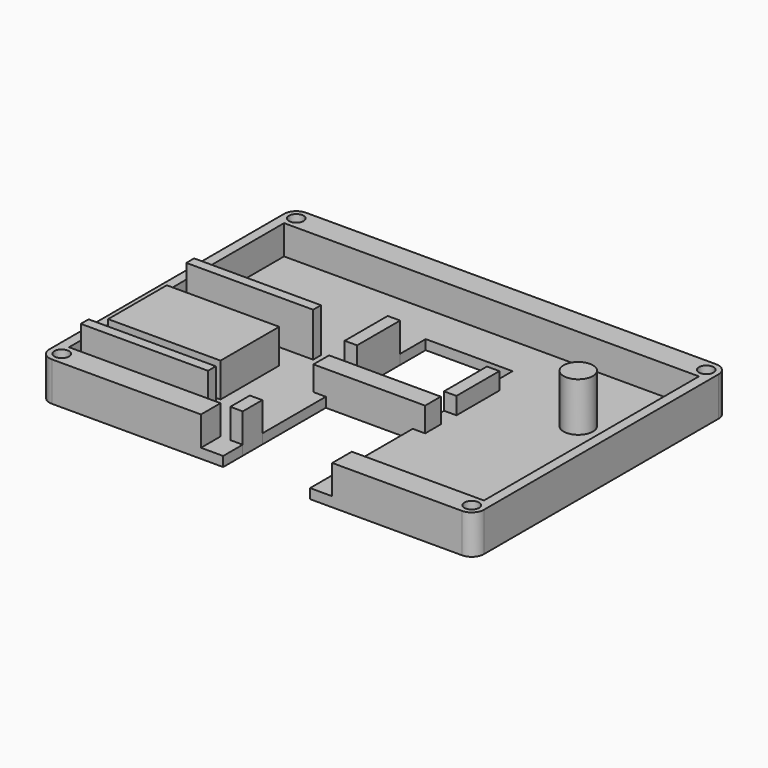
from build123d import *

# Parameters (mm, degrees)
F0_R     = 1.5
F1_DEPTH = 8
F0_W     = 2.54
F0_H     = 11
F0_H_2   = 5
F0_R_2   = 3
F0_H_3   = 16.26
F0_H_4   = 4
F2_DEPTH = 2
F0_W_2   = 23
F0_H_5   = 15
F3_DEPTH = 9
F0_W_3   = 25.9549565881
F0_H_6   = 2
F4_DEPTH = 11
F0_W_4   = 17.78
F5_DEPTH = 7
F6_DEPTH = 5.5
F7_DEPTH = 12


# Not quite as in the source:
# - a feature names something its author has since deleted; it is built from what else it names


with BuildPart() as f1:
    # F0 (on Top) → F1 (new body)
    with BuildSketch(Plane.XY):
        with BuildLine():
            Line((-42.45, 27.5), (42.45, 27.5))
            Line((42.45, 27.5), (42.45, 0.5))
            Line((42.45, 0.5), (42.45, -20.5))
            Line((42.45, -20.5), (42.45, -27.5))
            Line((42.45, -27.5), (15.41, -27.5))
            Line((15.41, -27.5), (15.41, -32.5))
            Line((15.41, -32.5), (41.95, -32.5))
            ThreePointArc((41.95, -32.5), (43.717766953, -31.767766953), (44.45, -30))
            Line((44.45, -30), (44.45, -27.5))
            Line((44.45, -27.5), (44.45, 27.5))
            Line((44.45, 27.5), (44.45, 30))
            ThreePointArc((44.45, 30), (43.717766953, 31.767766953), (41.95, 32.5))
            Line((41.95, 32.5), (-41.95, 32.5))
            ThreePointArc((-41.95, 32.5), (-43.717766953, 31.767766953), (-44.45, 30))
            Line((-44.45, 30), (-44.45, 27.5))
            Line((-44.45, 27.5), (-44.45, -27.5))
            Line((-44.45, -27.5), (-44.45, -30))
            ThreePointArc((-44.45, -30), (-43.717766953, -31.767766953), (-41.95, -32.5))
            Line((-41.95, -32.5), (-11.45, -32.5))
            Line((-11.45, -32.5), (-11.45, -27.5))
            Line((-11.45, -27.5), (-42.45, -27.5))
            Line((-42.45, -27.5), (-42.45, -24.5))
            Line((-42.45, -24.5), (-42.45, -22.5))
            Line((-42.45, -22.5), (-42.45, -20.5))
            Line((-42.45, -20.5), (-42.45, -17.5))
            Line((-42.45, -17.5), (-42.45, -2.5))
            Line((-42.45, -2.5), (-42.45, 0.5))
            Line((-42.45, 0.5), (-42.45, 2.5))
            Line((-42.45, 2.5), (-42.45, 4.5))
            Line((-42.45, 4.5), (-42.45, 27.5))
        make_face()
        with Locations((-41.95, -30)):
            Circle(F0_R, mode=Mode.SUBTRACT)
        with Locations((41.95, -30)):
            Circle(F0_R, mode=Mode.SUBTRACT)
        with Locations((-41.95, 30)):
            Circle(F0_R, mode=Mode.SUBTRACT)
        with Locations((41.95, 30)):
            Circle(F0_R, mode=Mode.SUBTRACT)
    extrude(amount=F1_DEPTH)

    # F0 (on Top) → F2 (join)
    with BuildSketch(Plane.XY):
        Polygon((42.45, 0.5), (42.45, 27.5), (-42.45, 27.5), (-42.45, 4.5), (-16.4950434119, 4.5), (-16.4950434119, 2.5), (-42.45, 2.5), (-42.45, 0.5), (-16.45, 0.5), (-16.45, -20.5), (-42.45, -20.5), (-42.45, -22.5), (-16.4950434119, -22.5), (-16.419, -22.5), (-16.419, -24.5), (-42.45, -24.5), (-42.45, -27.5), (-11.45, -27.5), (-11.45, -32.5), (-9.45, -32.5), (-9.45, -27.5), (-9.45, -22.5), (-9.45, -6.24), (-9.45, -2.24), (-9.45, 1.76), (-9.45, 12.76), (-9.45, 18.3), (-6.91, 18.3), (-6.91, 19.3), (10.87, 19.3), (10.87, 18.3), (13.41, 18.3), (13.41, 12.76), (13.41, 1.76), (13.41, -2.24), (13.41, -6.24), (13.41, -32.5), (15.41, -32.5), (15.41, -27.5), (42.45, -27.5), (42.45, -20.5), align=None)
        with Locations((30.95, 11)):
            Circle(F0_R_2, mode=Mode.SUBTRACT)
        Polygon((-16.45, 0.5), (-42.45, 0.5), (-42.45, -2.5), (-19.45, -2.5), (-19.45, -17.5), (-42.45, -17.5), (-42.45, -20.5), (-16.45, -20.5), align=None)
        with Locations((-8.18, -14.37)):
            Rectangle(F0_W, F0_H_3)
        with Locations((-8.18, -4.24)):
            Rectangle(F0_W, F0_H_4)
        with Locations((-8.18, -0.24)):
            Rectangle(F0_W, F0_H_4)
        Polygon((-9.45, 12.76), (-6.91, 12.76), (-6.91, 15.76), (-6.91, 18.3), (-9.45, 18.3), align=None)
        Polygon((-9.45, -32.5), (-6.91, -32.5), (-6.91, -29.96), (-6.91, -27.5), (-9.45, -27.5), align=None)
        Polygon((10.87, -32.5), (13.41, -32.5), (13.41, -6.24), (10.87, -6.24), (10.87, -29.96), align=None)
        with Locations((12.14, -4.24)):
            Rectangle(F0_W, F0_H_4)
        Polygon((10.87, 12.76), (13.41, 12.76), (13.41, 18.3), (10.87, 18.3), (10.87, 15.76), align=None)
        with Locations((12.14, -0.24)):
            Rectangle(F0_W, F0_H_4)
    extrude(amount=F2_DEPTH)

    # F0 (on Top) → F3 (join)
    with BuildSketch(Plane.XY):
        with Locations((-30.95, -10)):
            Rectangle(F0_W_2, F0_H_5)
    extrude(amount=F3_DEPTH)

    # F0 (on Top) → F4 (join)
    with BuildSketch(Plane.XY):
        with Locations((-29.4725217059, 3.5)):
            Rectangle(F0_W_3, F0_H_6)
        Polygon((-16.4950434119, -22.5), (-42.45, -22.5), (-42.45, -24.5), (-16.419, -24.5), (-16.419, -22.5), align=None)
    extrude(amount=F4_DEPTH)

    # F0 (on Top) → F5 (join)
    with BuildSketch(Plane.XY):
        with Locations((1.98, -4.24)):
            Rectangle(F0_W_4, F0_H_4)
        with Locations((12.14, -4.24)):
            Rectangle(F0_W, F0_H_4)
        with Locations((-8.18, -4.24)):
            Rectangle(F0_W, F0_H_4)
    extrude(amount=F5_DEPTH)

    # F0 (on Top) → F6 (join)
    with BuildSketch(Plane.XY):
        with Locations((12.14, 7.26)):
            Rectangle(F0_W, F0_H)
    extrude(amount=F6_DEPTH)

    # F0 (on Top) → F7 (join)
    with BuildSketch(Plane.XY):
        with Locations((30.95, 11)):
            Circle(F0_R_2)
    extrude(amount=F7_DEPTH)


with BuildPart() as f1b:
    # F0 (on Top) → F1, piece 2 (new body)
    with BuildSketch(Plane.XY):
        with Locations((-8.18, 7.26)):
            Rectangle(F0_W, F0_H)
    extrude(amount=F1_DEPTH)


with BuildPart() as f1c:
    # F0 (on Top) → F1, piece 3 (new body)
    with BuildSketch(Plane.XY):
        with Locations((-8.18, -25)):
            Rectangle(F0_W, F0_H_2)
    extrude(amount=F1_DEPTH)


solid = Compound([f1.part, f1b.part, f1c.part])
